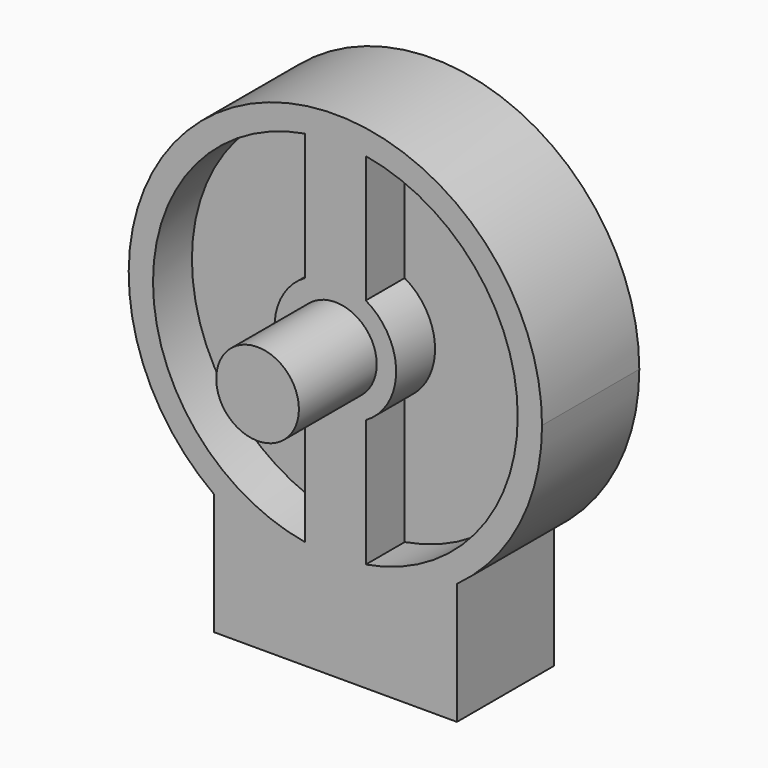
from build123d import *

# Parameters (mm, degrees)
F1_DEPTH = 10
F3_DEPTH = 4
F4_R     = 3.4
F5_DEPTH = 8


# Not quite as in the source:
# - a feature of the source that left no trace in its solid (it failed there, or was rolled back) is left out
# - a pattern or mirror of a feature is missing from the dataset's text; its kind, count and spacing are read off the source's solid


with BuildPart() as f1:
    # F0 (on Front) → F1 (new body)
    with BuildSketch(Plane.XZ):
        with BuildLine():
            ThreePointArc((10, -13.7477270849), (15.1492574075, -7.7136243103), (17, 0))
            ThreePointArc((17, 0), (-7.7136243103, 15.1492574075), (-10, -13.7477270849))
            ThreePointArc((-10, -13.7477270849), (0, -17), (10, -13.7477270849))
        make_face()
        with BuildLine():
            ThreePointArc((10, -13.7477270849), (0, -17), (-10, -13.7477270849))
            Line((-10, -13.7477270849), (-10, -23.7477270849))
            Line((-10, -23.7477270849), (10, -23.7477270849))
            Line((10, -23.7477270849), (10, -13.7477270849))
        make_face()
    extrude(amount=F1_DEPTH)

    # F2 (on face) → F3 (cut)
    with BuildSketch(Plane.XZ.offset(10)):
        with BuildLine():
            Line((-2.5, 4.3301270189), (-2.5, 14.7901994577))
            ThreePointArc((-2.5, 14.7901994577), (-15, 0), (-2.5, -14.7901994577))
            Line((-2.5, -14.7901994577), (-2.5, -4.3301270189))
            ThreePointArc((-2.5, -4.3301270189), (-5, 0), (-2.5, 4.3301270189))
        make_face()
    f3 = extrude(amount=-F3_DEPTH, mode=Mode.SUBTRACT)

    # F3_copies: F3 across plane
    add(f3.mirror(Plane(origin=(0, 0, 0), x_dir=(0, 0, 1), z_dir=(1, 0, 0))), mode=Mode.SUBTRACT)

    # F4 (on face) → F5 (join)
    with BuildSketch(Plane.XZ.offset(10)):
        Circle(F4_R)
    extrude(amount=F5_DEPTH)


solid = f1.part
